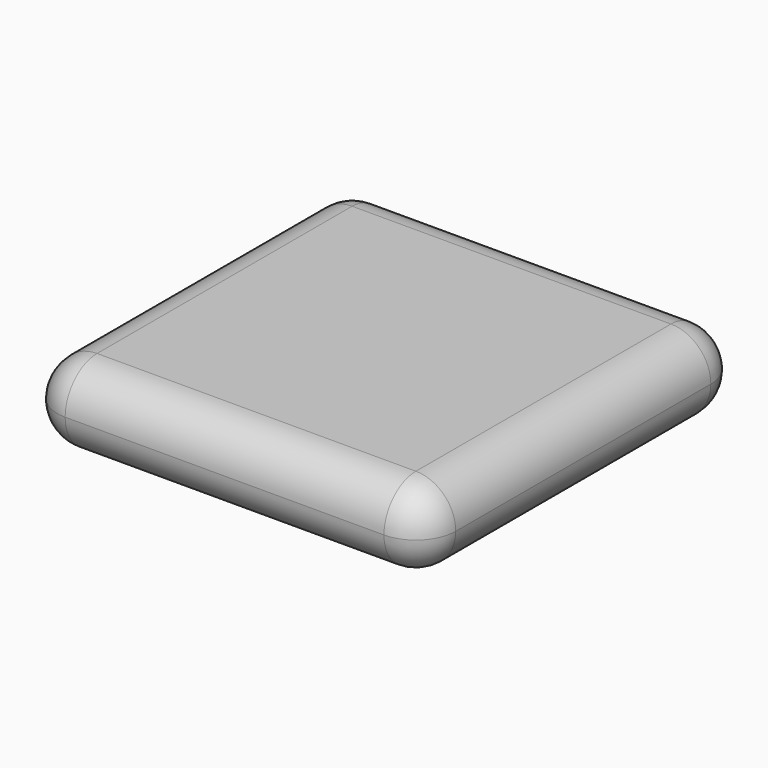
from build123d import *

# Parameters (mm, degrees)
F0_W     = 50
F0_H     = 50
F1_DEPTH = 10
F2_R     = 4.99999


# Not quite as in the source:
# - a fillet or chamfer is up to 0.001 mm smaller than in the source, because OpenCascade refuses the exact size


with BuildPart() as f1:
    # F0 (on Top) → F1 (new body)
    with BuildSketch(Plane.XY):
        Rectangle(F0_W, F0_H)
    extrude(amount=F1_DEPTH)

    # F2 (radius 5 in the source; OpenCascade refuses exactly that, so slightly less here)
    f2_edges = [f1.edges().sort_by_distance(p)[0] for p in [
        (-25, 0, 10),
        (-25, 0, 0),
        (0, -25, 0),
        (0, -25, 10),
        (-25, -25, 5),
        (25, -25, 5),
        (25, 0, 10),
        (25, 0, 0),
        (0, 25, 0),
        (0, 25, 10),
        (25, 25, 5),
        (-25, 25, 5),
    ]]
    fillet(f2_edges, radius=F2_R)


solid = f1.part
